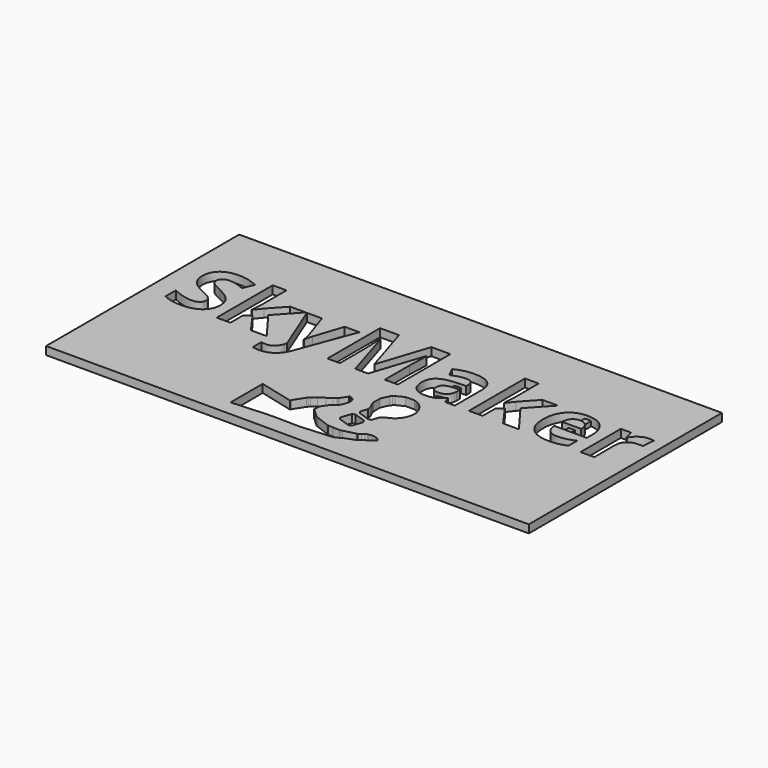
from build123d import *

# Parameters (mm, degrees)
F0_W         = 120
F0_H         = 60
F1_DEPTH     = 2
F2_TEXT_SIZE = 22.9166666667
F3_DEPTH     = 25
F5_DEPTH     = 25
F6_W         = 1.6
F6_H         = 10
F7_DEPTH     = 1.2


# Not quite as in the source:
# - Text() gives the source's letters only with a copy of the font that has no kerning and outlines rounded to 1/6400 em; it was checked with that copy


with BuildPart() as f1:
    # F0 (on Top) → F1 (new body)
    with BuildSketch(Plane.XY):
        with Locations((-1, 0)):
            Rectangle(F0_W, F0_H)
    extrude(amount=F1_DEPTH)

    # F2 (on face) → F3 (cut)
    with BuildSketch(Plane.XY.offset(2)):
        with Locations((-57, 0)):
            Text('SkyMaker', F2_TEXT_SIZE, font='Open Sans', font_style=FontStyle.BOLD, text_align=(TextAlign.LEFT, TextAlign.BOTTOM))
    extrude(amount=-F3_DEPTH, mode=Mode.SUBTRACT)

    # F4 (on face) → F5 (cut)
    with BuildSketch(Plane.XY.offset(2)):
        Polygon((-9.7223075204, -18.2968813044), (-18.2257756004, -16.1556778736), (-18.2257756004, -26.1556778736), (-16.9082824258, -26.0635886796), (-13.8179897491, -25.8640385162), (-10.2544255719, -25.6696279955), (-8.1439656918, -25.5826312915), (-7.5094791609, -25.5877709342), (-7.1692725379, -25.5877709342), (-6.1434187206, -25.6056418018), (-4.2657044942, -25.6414778425), (-2.4877181967, -25.6747204855), (-1.5872433692, -25.6849526182), (-1.4132971138, -25.6798601282), (-1.2137469505, -25.6721742405), (0.1139312042, -25.5698529138), (1.4262847362, -25.4521598118), (1.6181490119, -25.4393814341), (1.8074198899, -25.4240096588), (2.7233136455, -25.3779886381), (3.7517137077, -25.3191420871), (3.9998311368, -25.3012240667), (4.3298527798, -25.2731210664), (5.6191958015, -25.2193670054), (6.6194457107, -25.0607453727), (6.8036712514, -24.981481709), (6.9264568435, -24.9303210457), (7.5736274466, -24.5772888923), (8.3538629271, -24.1551780552), (8.5431809578, -24.0733209938), (8.8144032026, -23.9504882491), (9.8734996628, -23.54888883), (10.5974348373, -23.2981780033), (10.7048958067, -23.2495635849), (10.8097162257, -23.1984029216), (11.3725778278, -22.7916638598), (12.0991064, -22.236535298), (12.285831033, -22.1137025533), (12.4726028187, -21.9909169613), (13.4651668403, -21.4025457565), (14.0381662697, -20.9215883684), (14.0152029121, -20.8525568374), (13.9486704734, -20.6657850517), (13.539338014, -20.1874210612), (12.8000310641, -19.8830033262), (11.9123346143, -19.8394813978), (11.2190486851, -19.9213856118), (10.9939417664, -19.9674066325), (10.8506447563, -19.9955567855), (10.4490924899, -20.1950597962), (9.8760459078, -20.5711496127), (9.4232386727, -20.9241817661), (9.241559377, -21.0827562461), (8.9550596622, -21.1313706644), (6.1666384756, -21.8553529916), (5.8954633835, -21.9525346756), (5.5398849851, -21.9806848286), (3.9179740754, -21.942302543), (2.7053484724, -21.8860493896), (2.5595995228, -21.906513655), (2.2499949923, -21.7581241549), (-0.9502577461, -20.5813817453), (-1.2802793891, -20.4943850413), (-1.4030649812, -20.4150742249), (-2.4774860641, -19.4531594487), (-2.5670290131, -19.343199387), (-2.6514323194, -19.2382846627), (-3.6517293814, -18.3608674981), (-3.7668762384, -18.2917888145), (-3.672146494, -16.6672845071), (-2.4391037784, -14.899577495), (-2.3035398087, -14.8177204336), (-1.1140190214, -13.7740429014), (-1.0141967871, -13.6512573094), (-0.891411195, -13.4491137483), (-0.5921331027, -12.7993497475), (-0.3107258779, -11.8297490836), (-0.2953541026, -10.9114033884), (-0.5281940616, -10.3332643163), (-0.6663042763, -10.2130249692), (-0.8504826644, -10.0518570915), (-1.5411751959, -9.7397063161), (-1.8047115529, -9.8011462648), (-1.889162012, -9.9700000302), (-2.9098761865, -11.5508881039), (-3.0301155336, -11.6967785116), (-3.1938296563, -11.8809097469), (-3.8103510141, -12.3183923594), (-4.9717216483, -13.0398284416), (-6.342968884, -13.9658600244), (-7.4327145896, -14.863788607), (-7.75759659, -15.1989027401), (-7.967378886, -15.4240568115), (-9.6071606634, -18.0103815897), align=None)
        Polygon((6.240856802, -19.0592459173), (7.1080418338, -16.5240818024), (6.7601021704, -15.9254313122), (3.8514416367, -14.9328672907), (3.2042710336, -15.2526568011), (2.3447247367, -17.7775416306), (2.7462770031, -18.3505882128), (5.6294279341, -19.338106897), align=None)
        Polygon((10.4056177143, -11.7504382672), (10.541181684, -11.6813595836), (10.814903021, -11.5048670832), (11.5413844405, -10.8167207967), (12.25258839, -9.7269279385), (12.6388631864, -8.4861993352), (12.7053956251, -7.4884956709), (12.6670133394, -7.1636136705), (12.6260848088, -6.8387316701), (12.321619921, -5.8845499342), (11.6513916549, -4.7717465656), (10.7023495617, -3.8840029631), (9.8325711321, -3.3902671973), (9.5230137544, -3.2853524729), (9.0958104273, -3.1396035233), (6.9290030884, -3.1574743909), (4.9796167806, -4.1091098818), (4.6649669129, -4.4314456372), (4.3477708002, -4.7512351476), (3.4216920646, -6.7108064354), (3.4319241973, -8.8801600193), (3.5828599423, -9.3048171013), (3.6365668507, -9.4762642644), (3.723516402, -9.6911390505), (4.1993813001, -10.711853225), (4.3554566878, -11.7197418692), (4.2837846065, -11.932117563), (3.7926422384, -13.4056389727), (4.1968350551, -13.9812317998), (7.0108601498, -14.9635636887), (7.7271094366, -14.771699413), (8.2182989574, -13.2674816053), (8.2899710388, -13.0526068192), (9.0855311419, -12.3874710431), (10.1830098879, -11.8834559919), align=None)
    extrude(amount=-F5_DEPTH, mode=Mode.SUBTRACT)


with BuildPart() as f7:
    # F6 (on face) → F7 (new body)
    with BuildSketch(Plane(origin=(0, 0, 0), x_dir=(1, 0, 0), z_dir=(0, 0, -1))):
        with Locations((39.5362670153, -8.9476349056)):
            Rectangle(F6_W, F6_H)
    extrude(amount=-F7_DEPTH)


with BuildPart() as f7b:
    # F6 (on face) → F7, piece 2 (new body)
    with BuildSketch(Plane(origin=(0, 0, 0), x_dir=(1, 0, 0), z_dir=(0, 0, -1))):
        with Locations((11.1785596237, -3.7802795414)):
            Rectangle(F6_W, F6_H)
    extrude(amount=-F7_DEPTH)


solid = Compound([f1.part, f7.part, f7b.part])
